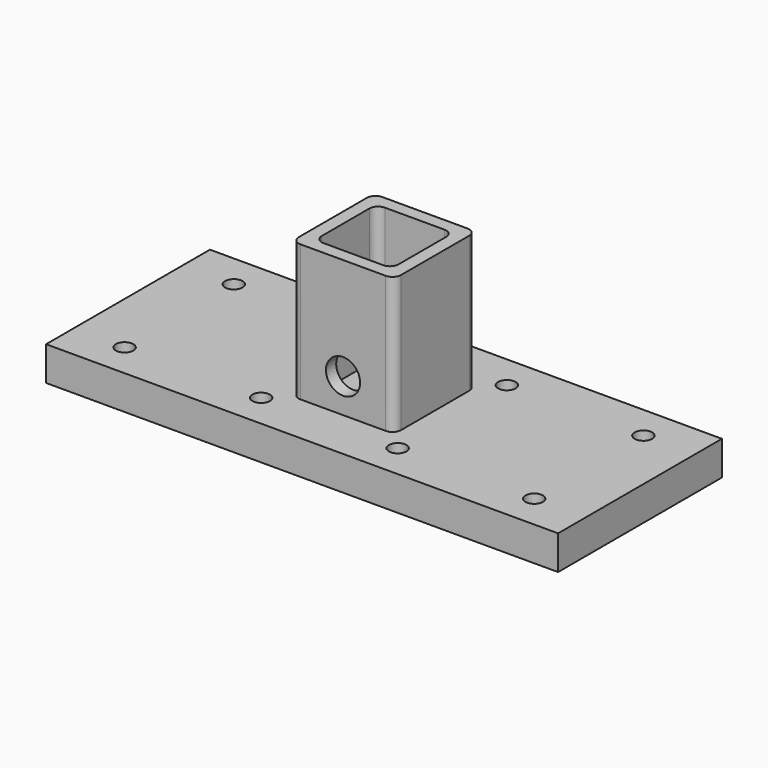
from build123d import *

# Parameters (mm, degrees)
F0_W     = 190.5
F0_H     = 76.2
F1_DEPTH = 6.35
F3_D     = 6.5278
F4_W     = 38.1
F4_H     = 38.1
F4_W_2   = 28.575
F4_H_2   = 28.575
F5_DEPTH = 50.8
F6_R     = 3.175
F7_R     = 6.35
F8_DEPTH = 38.1


# Not quite as in the source:
# - a feature names something its author has since deleted; it is built from what else it names


with BuildPart() as f1:
    # F0 (on Top) → F1 (new body, symmetric)
    with BuildSketch(Plane.XY):
        Rectangle(F0_W, F0_H)
    extrude(amount=F1_DEPTH, both=True)

    # F3 (through all)
    with Locations(Plane(origin=(0, 0, -6.35), x_dir=(1, 0, 0), z_dir=(0, 0, -1))):
        with Locations((-76.2, -25.4), (-25.4, -25.4), (-76.2, 25.4), (-25.4, 25.4), (25.4, 25.4), (25.4, -25.4), (76.2, -25.4), (76.2, 25.4)):
            Hole(F3_D / 2)

    # F4 (on face) → F5 (join)
    with BuildSketch(Plane.XY.offset(6.35)):
        Rectangle(F4_W, F4_H)
        Rectangle(F4_W_2, F4_H_2, mode=Mode.SUBTRACT)
    extrude(amount=F5_DEPTH)

    # F6
    f6_edges = [f1.edges().sort_by_distance(p)[0] for p in [
        (-19.05, -19.05, 31.75),
        (19.05, -19.05, 31.75),
        (-14.2875, 14.2875, 31.75),
        (14.2875, 14.2875, 31.75),
        (-14.2875, -14.2875, 31.75),
        (14.2875, -14.2875, 31.75),
        (-19.05, 19.05, 31.75),
        (19.05, 19.05, 31.75),
    ]]
    fillet(f6_edges, radius=F6_R)

    # F7 (on face) → F8 (cut, through all)
    with BuildSketch(Plane.XZ.offset(19.05)):
        with Locations((0, 19.05)):
            Circle(F7_R)
    extrude(amount=-F8_DEPTH, mode=Mode.SUBTRACT)


solid = f1.part
